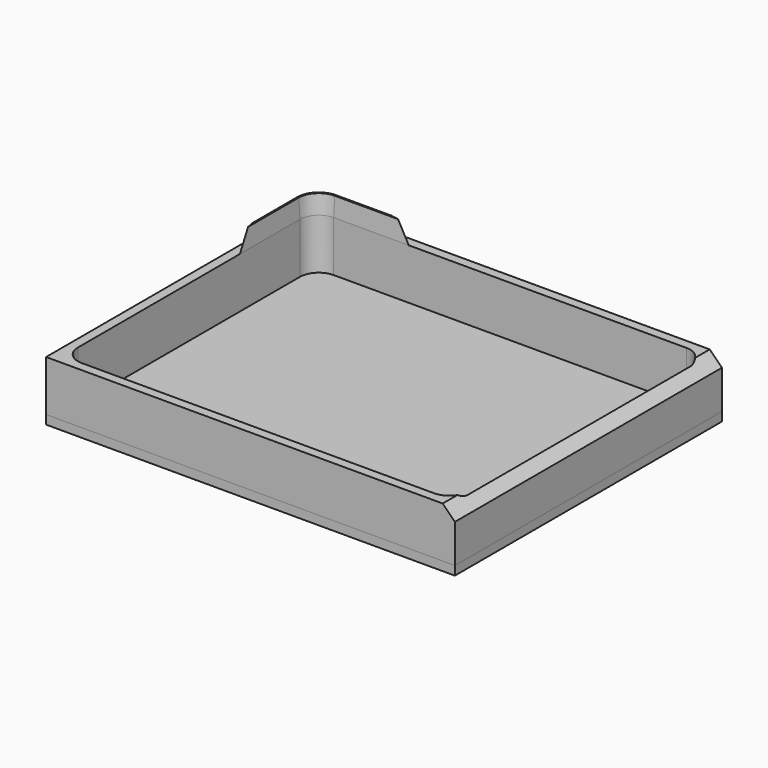
from build123d import *

# Parameters (mm, degrees)
F1_DEPTH    = 27
F2_T1_DEPTH = 211.4318788436
F3_DEPTH    = 4.7625
F5_DEPTH    = 10
F5_TAPER    = 3.5


# Not quite as in the source:
# - a fillet or chamfer that OpenCascade refuses, or shapes differently, is made with other operations: its cross-section is extruded or revolved along the edge and cut away or added
# - a length typed as a fraction of an inch, garbled in the dataset ("3 / 203.2 mm" for 3/8 in), is restored
# - a feature names something its author has since deleted; it is built from what else it names


with BuildPart() as f1:
    # F0 (on Top) → F1 (new body)
    with BuildSketch(Plane.XY):
        Polygon((-112.323590219, 87.2017167807), (-112.323590219, -90.7982832193), (105.676409781, -90.7982832193), (105.676409781, 77.2017167807), (105.676409781, 87.2017167807), align=None)
        with BuildLine():
            ThreePointArc((-107.323590219, 72.2017167807), (-104.3946580309, 79.2727845925), (-97.323590219, 82.2017167807))
            Line((-97.323590219, 82.2017167807), (90.676409781, 82.2017167807))
            ThreePointArc((90.676409781, 82.2017167807), (97.7474775928, 79.2727845925), (100.676409781, 72.2017167807))
            Line((100.676409781, 72.2017167807), (100.676409781, -75.7982832193))
            ThreePointArc((100.676409781, -75.7982832193), (97.7474775928, -82.8693510312), (90.676409781, -85.7982832193))
            Line((90.676409781, -85.7982832193), (-97.323590219, -85.7982832193))
            ThreePointArc((-97.323590219, -85.7982832193), (-104.3946580309, -82.8693510312), (-107.323590219, -75.7982832193))
            Line((-107.323590219, -75.7982832193), (-107.323590219, 72.2017167807))
        make_face(mode=Mode.SUBTRACT)
    extrude(amount=F1_DEPTH)

    # F2: chamfer of 6.5 on 1 edges, made by hand

    # F2_s2 → F2_t1 (cut)
    with BuildSketch(Plane.XZ.offset(-103.9176562024)):
        Polygon((99.176409781, 27), (105.676409781, 20.5), (105.676409781, 27), align=None)
    extrude(amount=F2_T1_DEPTH, mode=Mode.SUBTRACT)

    # F4 (on face) → F5 (join)
    with BuildSketch(Plane.XY.offset(27)):
        with BuildLine():
            ThreePointArc((-107.323590219, 72.2017167807), (-104.3946580309, 79.2727845925), (-97.323590219, 82.2017167807))
            Line((-97.323590219, 82.2017167807), (-57.323590219, 82.2017167807))
            Line((-57.323590219, 82.2017167807), (-67.323590219, 84.2017167807))
            Line((-67.323590219, 84.2017167807), (-97.323590219, 84.2017167807))
            ThreePointArc((-97.323590219, 84.2017167807), (-105.8088715933, 80.6869981549), (-109.323590219, 72.2017167807))
            Line((-109.323590219, 72.2017167807), (-109.323590219, 42.2017167807))
            Line((-109.323590219, 42.2017167807), (-107.323590219, 32.2017167807))
            Line((-107.323590219, 32.2017167807), (-107.323590219, 72.2017167807))
        make_face()
    extrude(amount=F5_DEPTH, taper=F5_TAPER)


with BuildPart() as f3:
    # F0 (on Top) → F3 (new body)
    with BuildSketch(Plane.XY):
        Polygon((-112.323590219, 87.2017167807), (-112.323590219, -90.7982832193), (105.676409781, -90.7982832193), (105.676409781, 77.2017167807), (105.676409781, 87.2017167807), align=None)
        with BuildLine():
            ThreePointArc((-107.323590219, 72.2017167807), (-104.3946580309, 79.2727845925), (-97.323590219, 82.2017167807))
            Line((-97.323590219, 82.2017167807), (90.676409781, 82.2017167807))
            ThreePointArc((90.676409781, 82.2017167807), (97.7474775928, 79.2727845925), (100.676409781, 72.2017167807))
            Line((100.676409781, 72.2017167807), (100.676409781, -75.7982832193))
            ThreePointArc((100.676409781, -75.7982832193), (97.7474775928, -82.8693510312), (90.676409781, -85.7982832193))
            Line((90.676409781, -85.7982832193), (-97.323590219, -85.7982832193))
            ThreePointArc((-97.323590219, -85.7982832193), (-104.3946580309, -82.8693510312), (-107.323590219, -75.7982832193))
            Line((-107.323590219, -75.7982832193), (-107.323590219, 72.2017167807))
        make_face(mode=Mode.SUBTRACT)
        with BuildLine():
            Line((90.676409781, 82.2017167807), (-97.323590219, 82.2017167807))
            ThreePointArc((-97.323590219, 82.2017167807), (-104.3946580309, 79.2727845925), (-107.323590219, 72.2017167807))
            Line((-107.323590219, 72.2017167807), (-107.323590219, -75.7982832193))
            ThreePointArc((-107.323590219, -75.7982832193), (-104.3946580309, -82.8693510312), (-97.323590219, -85.7982832193))
            Line((-97.323590219, -85.7982832193), (90.676409781, -85.7982832193))
            ThreePointArc((90.676409781, -85.7982832193), (97.7474775928, -82.8693510312), (100.676409781, -75.7982832193))
            Line((100.676409781, -75.7982832193), (100.676409781, 72.2017167807))
            ThreePointArc((100.676409781, 72.2017167807), (97.7474775928, 79.2727845925), (90.676409781, 82.2017167807))
        make_face()
    extrude(amount=-F3_DEPTH)


solid = Compound([f1.part, f3.part])
